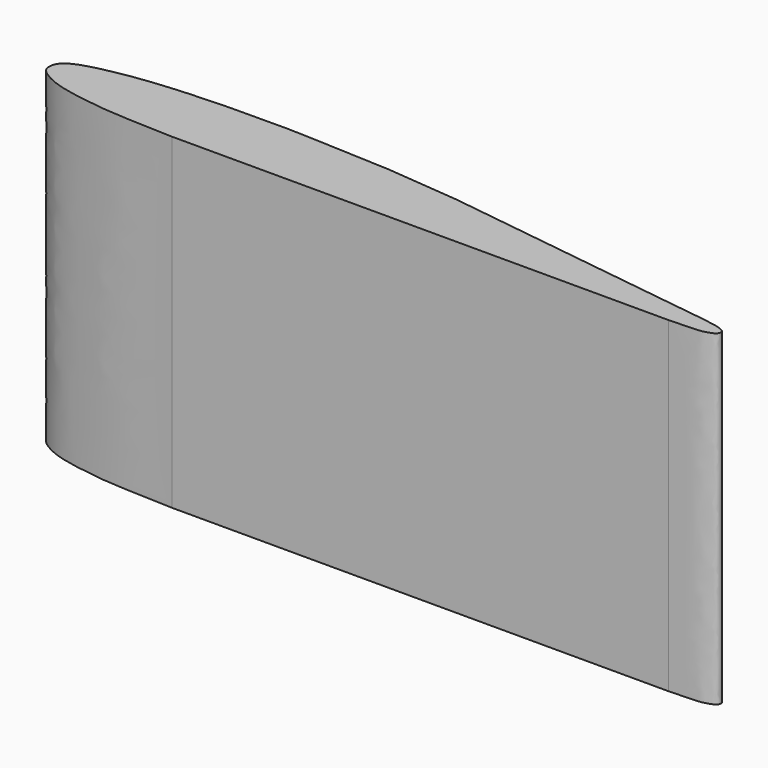
from build123d import *

# Parameters (mm, degrees)
F1_DEPTH = 25


# Not quite as in the source:
# - a feature names something its author has since deleted; it is built from what else it names


with BuildPart() as f1:
    # F0 (on Top) → F1 (new body)
    with BuildSketch(Plane.XY):
        with BuildLine():
            add(Edge.make_bspline(
                [(20.717319, 0.961567), (20.732388, 0.950862), (20.802589, 0.89602), (20.844955, 0.835309), (20.868742, 0.786923)],
                knots=[0.900505, 0.900505, 0.900505, 0.900505, 0.902591, 0.910976, 0.910976, 0.910976, 0.910976], degree=3))
            add(Edge.make_bspline(
                [(20.868742, 0.786923), (20.868138, 0.789586), (20.854687, 0.844817), (20.81056, 0.907228), (20.741469, 0.948907), (20.717319, 0.961567)],
                knots=[0.615453, 0.615453, 0.615453, 0.615453, 0.618302, 0.675124, 0.702237, 0.702237, 0.702237, 0.702237], degree=3))
        make_face()
        with BuildLine():
            add(Edge.make_bspline(
                [(-20.564435, 0), (-22.194552, 0.095916), (-24.427051, 0.112259), (-26.507753, 0.301362), (-28.764397, 0.643243), (-30.183683, 1.005133), (-31.076947, 1.430682), (-31.969357, 2.019518), (-31.964602, 2.881289), (-31.272408, 3.798841), (-28.947606, 4.300063), (-27.40678, 4.550377)],
                knots=[0, 0, 0, 0, 0.065741, 0.112925, 0.162507, 0.202276, 0.235211, 0.267886, 0.295589, 0.330111, 0.386778, 0.386778, 0.386778, 0.386778], degree=3))
            Line((-20.564435, 0), (17.43832, 0))
            add(Edge.make_bspline(
                [(17.43832, 0), (18.30297, 0.017386), (19.576028, 0.042994), (20.126231, 0.173998), (20.550651, 0.314443), (20.758201, 0.42436), (20.871656, 0.585697), (20.881973, 0.728581), (20.868742, 0.786923)],
                knots=[0, 0, 0, 0, 0.216708, 0.324575, 0.419398, 0.489507, 0.553036, 0.615453, 0.615453, 0.615453, 0.615453], degree=3))
            add(Edge.make_bspline(
                [(20.717319, 0.961567), (20.732388, 0.950862), (20.802589, 0.89602), (20.844955, 0.835309), (20.868742, 0.786923)],
                knots=[0.900505, 0.900505, 0.900505, 0.900505, 0.902591, 0.910976, 0.910976, 0.910976, 0.910976], degree=3))
            add(Edge.make_bspline(
                [(20.717319, 0.961567), (20.683018, 0.979549), (20.544008, 1.039404), (20.237766, 1.203734), (19.221472, 1.343953), (19.235892, 1.357829)],
                knots=[0.702237, 0.702237, 0.702237, 0.702237, 0.740748, 0.843128, 0.984245, 0.984245, 0.984245, 0.984245], degree=3))
            add(Edge.make_bspline(
                [(19.224455, 1.359564), (19.228273, 1.358986), (19.232085, 1.358408), (19.235892, 1.357829)],
                knots=[0.866682, 0.866682, 0.866682, 0.866682, 0.866861, 0.866861, 0.866861, 0.866861], degree=3))
            add(Edge.make_bspline(
                [(17.149048, 1.638837), (17.932756, 1.531801), (18.641229, 1.447844), (19.224455, 1.359564)],
                knots=[0.839269, 0.839269, 0.839269, 0.839269, 0.866682, 0.866682, 0.866682, 0.866682], degree=3))
            Line((17.149048, 1.638837), (-2.194774, 4.262684))
            Line((-2.194774, 4.262684), (-7.739238, 4.77529))
            add(Edge.make_bspline(
                [(-13.688116, 5.043835), (-10.617589, 4.926011), (-7.713727, 4.770205), (-7.739238, 4.77529)],
                knots=[0.682499, 0.682499, 0.682499, 0.682499, 0.978368, 0.978368, 0.978368, 0.978368], degree=3))
            add(Edge.make_bspline(
                [(-15.810056, 5.116998), (-15.116587, 5.096277), (-14.397899, 5.071071), (-13.688116, 5.043835)],
                knots=[0.614106, 0.614106, 0.614106, 0.614106, 0.682499, 0.682499, 0.682499, 0.682499], degree=3))
            add(Edge.make_bspline(
                [(-20.307882, 5.086518), (-19.759765, 5.098118), (-18.786684, 5.118038), (-17.645973, 5.120053), (-17.57649, 5.103397), (-16.725493, 5.130724), (-15.810056, 5.116998)],
                knots=[0, 0, 0, 0, 0.235949, 0.418843, 0.463394, 0.707258, 0.707258, 0.707258, 0.707258], degree=3))
            Line((-20.307882, 5.086518), (-23.17922, 4.966494))
            add(Edge.make_bspline(
                [(-24.460868, 4.878573), (-24.03409, 4.904099), (-23.606993, 4.932384), (-23.17922, 4.966494)],
                knots=[0.103012, 0.103012, 0.103012, 0.103012, 0.21756, 0.21756, 0.21756, 0.21756], degree=3))
            add(Edge.make_bspline(
                [(-27.40678, 4.550377), (-27.039132, 4.595793), (-26.336936, 4.681227), (-25.451565, 4.814667), (-24.796358, 4.853182), (-24.460868, 4.878573)],
                knots=[0, 0, 0, 0, 0.348839, 0.666199, 1, 1, 1, 1], degree=3))
        make_face()
    extrude(amount=F1_DEPTH)


solid = f1.part
